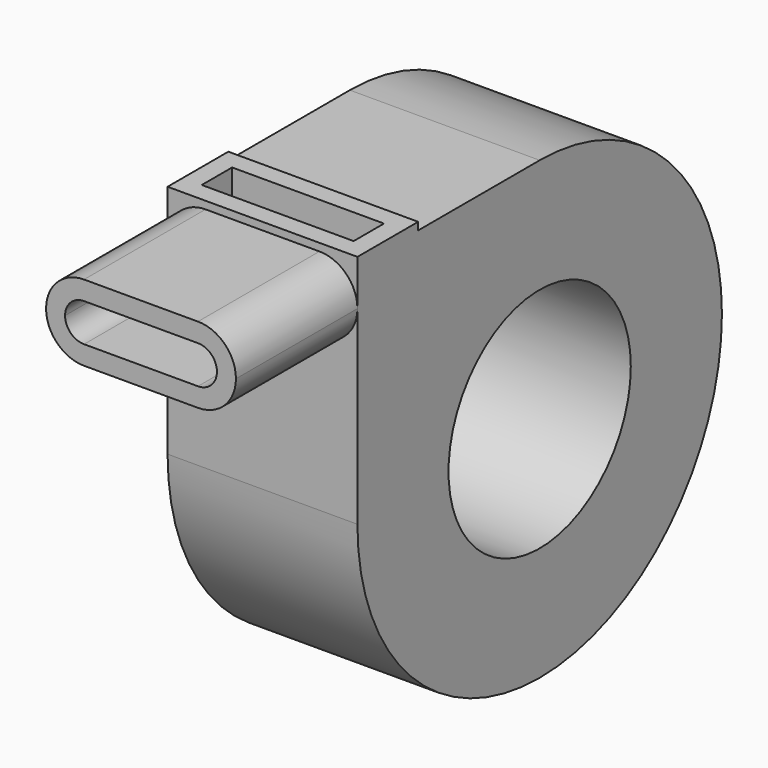
from build123d import *

# Parameters (mm, degrees)
F0_R     = 7.62
F0_W     = 5.08
F0_H     = 0.508
F1_DEPTH = 6.35
F2_T     = -1.27
F3_R     = 2.53999
F4_R     = 1.26999


# Not quite as in the source:
# - a fillet or chamfer is up to 0.001 mm smaller than in the source, because OpenCascade refuses the exact size


with BuildPart() as f1:
    # F0 (on Right) → F1 (new body, symmetric)
    with BuildSketch(Plane.YZ):
        with BuildLine():
            Line((-15.24, 15.24), (-25.4, 15.24))
            Line((-25.4, 15.24), (-25.4, 10.16))
            Line((-25.4, 10.16), (-15.24, 10.16))
            Line((-15.24, 10.16), (-15.24, 0))
            ThreePointArc((-15.24, 0), (10.7763073453, -10.7763073453), (0, 15.24))
            Line((0, 15.24), (-10.16, 15.24))
            Line((-10.16, 15.24), (-15.24, 15.24))
        make_face()
        Circle(F0_R, mode=Mode.SUBTRACT)
        with Locations((-12.7, 15.494)):
            Rectangle(F0_W, F0_H)
    extrude(amount=F1_DEPTH, both=True)

    # F2
    f2_openings = [f1.faces().sort_by_distance(p)[0] for p in [
        (0, -25.4, 12.7),
        (0, -12.7, 15.748),
    ]]
    offset(amount=F2_T, openings=f2_openings, kind=Kind.INTERSECTION)

    # F3 (radius 2.54 in the source; OpenCascade refuses exactly that, so slightly less here)
    f3_edges = [f1.edges().sort_by_distance(p)[0] for p in [
        (-6.35, -20.32, 15.24),
        (-6.35, -20.32, 10.16),
        (6.35, -20.32, 15.24),
        (6.35, -20.32, 10.16),
    ]]
    fillet(f3_edges, radius=F3_R)

    # F4 (radius 1.27 in the source; OpenCascade refuses exactly that, so slightly less here)
    f4_edges = [f1.edges().sort_by_distance(p)[0] for p in [
        (-5.08, -19.685, 11.43),
        (-5.08, -19.685, 13.97),
        (5.08, -19.685, 13.97),
        (5.08, -19.685, 11.43),
    ]]
    fillet(f4_edges, radius=F4_R)


solid = f1.part
